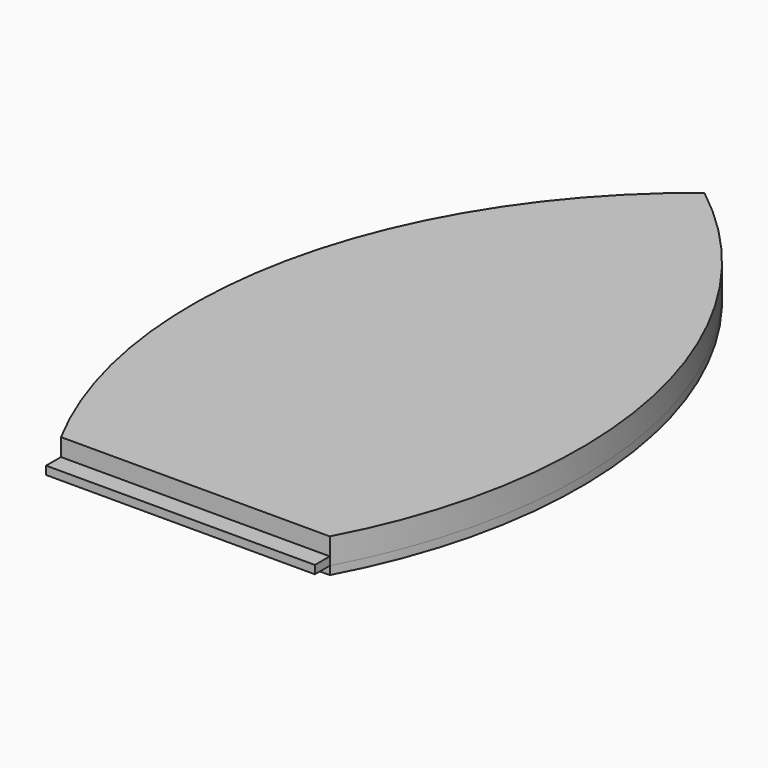
from build123d import *

# Parameters (mm, degrees)
F1_DEPTH = 8
F2_DEPTH = 25
F0_W     = 260.0473753379
F0_H     = 18
F3_DEPTH = 8


with BuildPart() as f1:
    # F0 (on Top) → F1 (new body, symmetric)
    with BuildSketch(Plane.XY):
        with BuildLine():
            ThreePointArc((130.023687669, -230.7024664879), (177.4658542143, 100.8481931393), (0, 384.8947908195))
            ThreePointArc((0, 384.8947908195), (-177.4658542143, 100.8481931393), (-130.023687669, -230.7024664879))
            Line((-130.023687669, -230.7024664879), (130.023687669, -230.7024664879))
        make_face()
        with BuildLine():
            ThreePointArc((-116.4091368779, -190.7024664879), (0, -46.4394716511), (116.4091368779, -190.7024664879))
            Line((116.4091368779, -190.7024664879), (-116.4091368779, -190.7024664879))
        make_face(mode=Mode.SUBTRACT)
        with BuildLine():
            ThreePointArc((-157.9683795481, 5.3817593866), (-147.7770049437, 96.2276147666), (-119.7465449836, 183.2398373016))
            ThreePointArc((-119.7465449836, 183.2398373016), (-106.6376449739, 190.2516231903), (-96.768933689, 179.1333077427))
            ThreePointArc((-96.768933689, 179.1333077427), (-84.7015708466, 105.2542818333), (-57.6378772255, 35.4596674073))
            ThreePointArc((-57.6378772255, 35.4596674073), (-90.8551676662, -36.1123876178), (-157.9683795481, 5.3817593866))
        make_face(mode=Mode.SUBTRACT)
        with BuildLine():
            ThreePointArc((0.1221596343, -14.9443653121), (-67.2509481397, 184.7158011806), (-0.2885299828, 384.5140801762))
            Line((-0.2885299828, 384.5140801762), (0.2888961989, 384.5140801762))
            ThreePointArc((0.2888961989, 384.5140801762), (67.3732536733, 184.7568211845), (0.1221596342, -14.9443653121))
        make_face(mode=Mode.SUBTRACT)
        with BuildLine():
            ThreePointArc((57.6378772255, 35.4596674073), (84.7015708466, 105.2542818333), (96.768933689, 179.1333077427))
            ThreePointArc((96.768933689, 179.1333077427), (106.6376449739, 190.2516231903), (119.7465449836, 183.2398373016))
            ThreePointArc((119.7465449836, 183.2398373016), (147.7770049437, 96.2276147666), (157.9683795481, 5.3817593866))
            ThreePointArc((157.9683795481, 5.3817593866), (90.8551676662, -36.1123876178), (57.6378772255, 35.4596674073))
        make_face(mode=Mode.SUBTRACT)
    extrude(amount=F1_DEPTH, both=True)


with BuildPart() as f2:
    # F0 (on Top) → F2 (new body)
    with BuildSketch(Plane.XY):
        with BuildLine():
            ThreePointArc((130.023687669, -230.7024664879), (177.4658542143, 100.8481931393), (0, 384.8947908195))
            ThreePointArc((0, 384.8947908195), (-177.4658542143, 100.8481931393), (-130.023687669, -230.7024664879))
            Line((-130.023687669, -230.7024664879), (130.023687669, -230.7024664879))
        make_face()
        with BuildLine():
            ThreePointArc((-116.4091368779, -190.7024664879), (0, -46.4394716511), (116.4091368779, -190.7024664879))
            Line((116.4091368779, -190.7024664879), (-116.4091368779, -190.7024664879))
        make_face(mode=Mode.SUBTRACT)
        with BuildLine():
            ThreePointArc((-157.9683795481, 5.3817593866), (-147.7770049437, 96.2276147666), (-119.7465449836, 183.2398373016))
            ThreePointArc((-119.7465449836, 183.2398373016), (-106.6376449739, 190.2516231903), (-96.768933689, 179.1333077427))
            ThreePointArc((-96.768933689, 179.1333077427), (-84.7015708466, 105.2542818333), (-57.6378772255, 35.4596674073))
            ThreePointArc((-57.6378772255, 35.4596674073), (-90.8551676662, -36.1123876178), (-157.9683795481, 5.3817593866))
        make_face(mode=Mode.SUBTRACT)
        with BuildLine():
            ThreePointArc((0.1221596343, -14.9443653121), (-67.2509481397, 184.7158011806), (-0.2885299828, 384.5140801762))
            Line((-0.2885299828, 384.5140801762), (0.2888961989, 384.5140801762))
            ThreePointArc((0.2888961989, 384.5140801762), (67.3732536733, 184.7568211845), (0.1221596342, -14.9443653121))
        make_face(mode=Mode.SUBTRACT)
        with BuildLine():
            ThreePointArc((57.6378772255, 35.4596674073), (84.7015708466, 105.2542818333), (96.768933689, 179.1333077427))
            ThreePointArc((96.768933689, 179.1333077427), (106.6376449739, 190.2516231903), (119.7465449836, 183.2398373016))
            ThreePointArc((119.7465449836, 183.2398373016), (147.7770049437, 96.2276147666), (157.9683795481, 5.3817593866))
            ThreePointArc((157.9683795481, 5.3817593866), (90.8551676662, -36.1123876178), (57.6378772255, 35.4596674073))
        make_face(mode=Mode.SUBTRACT)
        with BuildLine():
            Line((-116.4091368779, -190.7024664879), (116.4091368779, -190.7024664879))
            ThreePointArc((116.4091368779, -190.7024664879), (0, -46.4394716511), (-116.4091368779, -190.7024664879))
        make_face()
        with BuildLine():
            ThreePointArc((-96.768933689, 179.1333077427), (-106.6376449739, 190.2516231903), (-119.7465449836, 183.2398373016))
            ThreePointArc((-119.7465449836, 183.2398373016), (-147.7770049437, 96.2276147666), (-157.9683795481, 5.3817593866))
            ThreePointArc((-157.9683795481, 5.3817593866), (-90.8551676662, -36.1123876178), (-57.6378772255, 35.4596674073))
            ThreePointArc((-57.6378772255, 35.4596674073), (-84.7015708466, 105.2542818333), (-96.768933689, 179.1333077427))
        make_face()
        with BuildLine():
            Line((0.2888961989, 384.5140801762), (-0.2885299828, 384.5140801762))
            ThreePointArc((-0.2885299828, 384.5140801762), (-67.2509481397, 184.7158011806), (0.1221596343, -14.9443653121))
            ThreePointArc((0.1221596342, -14.9443653121), (67.3732536733, 184.7568211845), (0.2888961989, 384.5140801762))
        make_face()
        with BuildLine():
            ThreePointArc((0, 5.4204641238), (-55.3732812405, 184.8947908195), (0, 364.3691175153))
            ThreePointArc((0, 364.3691175153), (55.3732812405, 184.8947908195), (0, 5.4204641238))
        make_face(mode=Mode.SUBTRACT)
        with BuildLine():
            ThreePointArc((0, 5.4204641238), (55.3732812405, 184.8947908195), (0, 364.3691175153))
            ThreePointArc((0, 364.3691175153), (-55.3732812405, 184.8947908195), (0, 5.4204641238))
        make_face()
        with BuildLine():
            ThreePointArc((119.7465449836, 183.2398373016), (106.6376449739, 190.2516231903), (96.768933689, 179.1333077427))
            ThreePointArc((96.768933689, 179.1333077427), (84.7015708466, 105.2542818333), (57.6378772255, 35.4596674073))
            ThreePointArc((57.6378772255, 35.4596674073), (90.8551676662, -36.1123876178), (157.9683795481, 5.3817593866))
            ThreePointArc((157.9683795481, 5.3817593866), (147.7770049437, 96.2276147666), (119.7465449836, 183.2398373016))
        make_face()
    extrude(amount=F2_DEPTH)

    # F0 (on Top) → F3 (join)
    with BuildSketch(Plane.XY):
        with Locations((0, -239.7024664879)):
            Rectangle(F0_W, F0_H)
    extrude(amount=F3_DEPTH)


solid = Compound([f1.part, f2.part])
